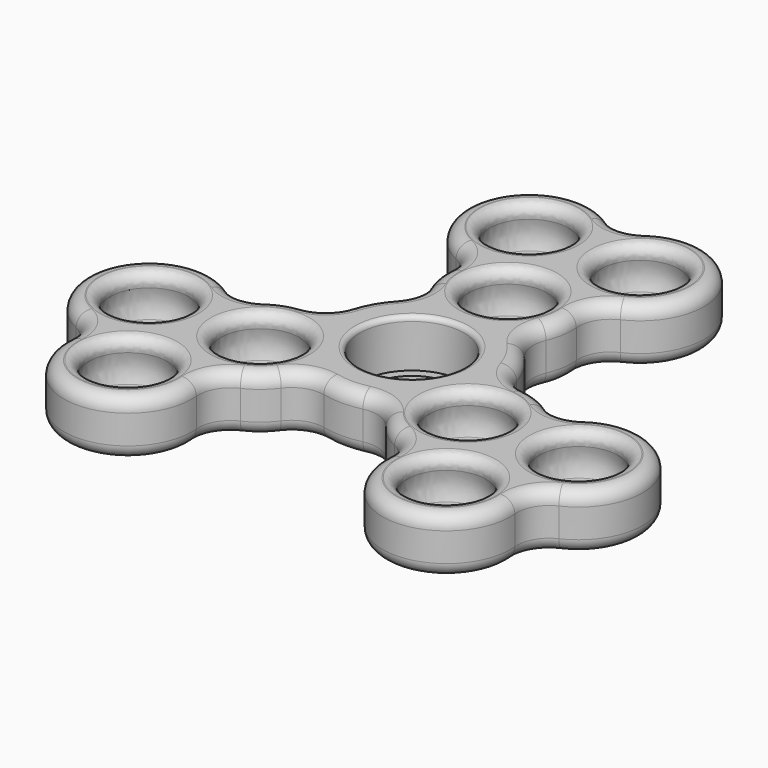
from build123d import *

# Parameters (mm, degrees)
F0_R      = 2.5
F0_R_2    = 6.525
F1_DEPTH  = 3.5
F2_DEPTH  = 3.5
F22_R     = 6.525
F22_R_2   = 5.3868073657
F23_DEPTH = 1
F24_R     = 1.7
F25_R     = 0.6
F26_R     = 1.32


with BuildPart() as f1:
    # F0 (on Top) → F1 (new body)
    with BuildSketch(Plane.XY):
        with BuildLine():
            ThreePointArc((62.7314133809, 3.8498463921), (61.4608563371, 1.9491717883), (59.3567896921, 1.0548660774))
            ThreePointArc((59.3567896921, 1.0548660774), (57.405087647, 0.5815289515), (55.6327668025, -0.3629644217))
            ThreePointArc((55.6327668025, -0.3629644217), (53.3233657257, -1.096978098), (51.0139646489, -0.3629644217))
            ThreePointArc((51.0139646489, -0.3629644217), (39.4669592652, -2.8949370692), (43.0477093227, -14.1609233929))
            ThreePointArc((43.0477093227, -14.1609233929), (44.8380843515, -15.7939165547), (45.3571103995, -18.1609233929))
            ThreePointArc((45.3571103995, -18.1609233929), (53.3233657257, -26.8949370692), (61.289621052, -18.1609233929))
            ThreePointArc((61.289621052, -18.1609233929), (61.8086470999, -15.7939165547), (63.5990221287, -14.1609233929))
            ThreePointArc((63.5990221287, -14.1609233929), (65.3031378059, -13.0982952045), (66.6889108041, -11.6447402157))
            ThreePointArc((66.6889108041, -11.6447402157), (68.5154355909, -10.2697179054), (70.796746604, -10.1197205304))
            ThreePointArc((70.796746604, -10.1197205304), (73.2419500127, -10.3949370692), (75.6871534215, -10.1197205304))
            ThreePointArc((75.6871534215, -10.1197205304), (77.9684644346, -10.2697179054), (79.7949892214, -11.6447402157))
            ThreePointArc((79.7949892214, -11.6447402157), (81.1807622196, -13.0982952045), (82.8848778968, -14.1609233929))
            ThreePointArc((82.8848778968, -14.1609233929), (84.6752529255, -15.7939165547), (85.1942789735, -18.1609233929))
            ThreePointArc((85.1942789735, -18.1609233929), (93.1605342998, -26.8949370692), (101.126789626, -18.1609233929))
            ThreePointArc((101.126789626, -18.1609233929), (101.645815674, -15.7939165547), (103.4361907028, -14.1609233929))
            ThreePointArc((103.4361907028, -14.1609233929), (107.0169407603, -2.8949370692), (95.4699353765, -0.3629644217))
            ThreePointArc((95.4699353765, -0.3629644217), (93.1605342998, -1.096978098), (90.851133223, -0.3629644217))
            ThreePointArc((90.851133223, -0.3629644217), (89.0788123785, 0.5815289515), (87.1271103334, 1.0548660774))
            ThreePointArc((87.1271103334, 1.0548660774), (85.0230436884, 1.9491717883), (83.7524866446, 3.8498463921))
            ThreePointArc((83.7524866446, 3.8498463921), (82.7682294544, 6.1050629308), (81.3072832359, 8.0850629308))
            ThreePointArc((81.3072832359, 8.0850629308), (80.2965292666, 10.1357349096), (80.5740711247, 12.4050629308))
            ThreePointArc((80.5740711247, 12.4050629308), (81.1400001716, 14.3319550455), (81.208205339, 16.3390766071))
            ThreePointArc((81.208205339, 16.3390766071), (81.727231387, 18.7060834453), (83.5176064158, 20.3390766071))
            ThreePointArc((83.5176064158, 20.3390766071), (87.0983564733, 31.6050629308), (75.5513510895, 34.1370355783))
            ThreePointArc((75.5513510895, 34.1370355783), (73.2419500127, 33.403021902), (70.932548936, 34.1370355783))
            ThreePointArc((70.932548936, 34.1370355783), (59.3855435522, 31.6050629308), (62.9662936097, 20.3390766071))
            ThreePointArc((62.9662936097, 20.3390766071), (64.7566686385, 18.7060834453), (65.2756946865, 16.3390766071))
            ThreePointArc((65.2756946865, 16.3390766071), (65.3438998539, 14.3319550455), (65.9098289008, 12.4050629308))
            ThreePointArc((65.9098289008, 12.4050629308), (66.1873707589, 10.1357349096), (65.1766167896, 8.0850629308))
            ThreePointArc((65.1766167896, 8.0850629308), (63.7156705711, 6.1050629308), (62.7314133809, 3.8498463921))
        make_face()
        with Locations((53.3233657257, -18.8949370692)):
            Circle(F0_R, mode=Mode.SUBTRACT)
        with Locations((46.3951624954, -6.8949370692)):
            Circle(F0_R, mode=Mode.SUBTRACT)
        with Locations((60.251568956, -6.8949370692)):
            Circle(F0_R, mode=Mode.SUBTRACT)
        with Locations((73.2419500127, 0.6050629308)):
            Circle(F0_R_2, mode=Mode.SUBTRACT)
        with Locations((93.1605342998, -18.8949370692)):
            Circle(F0_R, mode=Mode.SUBTRACT)
        with Locations((86.2323310695, -6.8949370692)):
            Circle(F0_R, mode=Mode.SUBTRACT)
        with Locations((100.0887375301, -6.8949370692)):
            Circle(F0_R, mode=Mode.SUBTRACT)
        with Locations((73.2419500127, 15.6050629308)):
            Circle(F0_R, mode=Mode.SUBTRACT)
        with Locations((66.3137467825, 27.6050629308)):
            Circle(F0_R, mode=Mode.SUBTRACT)
        with Locations((80.170153243, 27.6050629308)):
            Circle(F0_R, mode=Mode.SUBTRACT)
    extrude(amount=F1_DEPTH)

    # F0 (on Top) → F2 (join)
    with BuildSketch(Plane.XY):
        with BuildLine():
            ThreePointArc((62.7314133809, 3.8498463921), (61.4608563371, 1.9491717883), (59.3567896921, 1.0548660774))
            ThreePointArc((59.3567896921, 1.0548660774), (57.405087647, 0.5815289515), (55.6327668025, -0.3629644217))
            ThreePointArc((55.6327668025, -0.3629644217), (53.3233657257, -1.096978098), (51.0139646489, -0.3629644217))
            ThreePointArc((51.0139646489, -0.3629644217), (39.4669592652, -2.8949370692), (43.0477093227, -14.1609233929))
            ThreePointArc((43.0477093227, -14.1609233929), (44.8380843515, -15.7939165547), (45.3571103995, -18.1609233929))
            ThreePointArc((45.3571103995, -18.1609233929), (53.3233657257, -26.8949370692), (61.289621052, -18.1609233929))
            ThreePointArc((61.289621052, -18.1609233929), (61.8086470999, -15.7939165547), (63.5990221287, -14.1609233929))
            ThreePointArc((63.5990221287, -14.1609233929), (65.3031378059, -13.0982952045), (66.6889108041, -11.6447402157))
            ThreePointArc((66.6889108041, -11.6447402157), (68.5154355909, -10.2697179054), (70.796746604, -10.1197205304))
            ThreePointArc((70.796746604, -10.1197205304), (73.2419500127, -10.3949370692), (75.6871534215, -10.1197205304))
            ThreePointArc((75.6871534215, -10.1197205304), (77.9684644346, -10.2697179054), (79.7949892214, -11.6447402157))
            ThreePointArc((79.7949892214, -11.6447402157), (81.1807622196, -13.0982952045), (82.8848778968, -14.1609233929))
            ThreePointArc((82.8848778968, -14.1609233929), (84.6752529255, -15.7939165547), (85.1942789735, -18.1609233929))
            ThreePointArc((85.1942789735, -18.1609233929), (93.1605342998, -26.8949370692), (101.126789626, -18.1609233929))
            ThreePointArc((101.126789626, -18.1609233929), (101.645815674, -15.7939165547), (103.4361907028, -14.1609233929))
            ThreePointArc((103.4361907028, -14.1609233929), (107.0169407603, -2.8949370692), (95.4699353765, -0.3629644217))
            ThreePointArc((95.4699353765, -0.3629644217), (93.1605342998, -1.096978098), (90.851133223, -0.3629644217))
            ThreePointArc((90.851133223, -0.3629644217), (89.0788123785, 0.5815289515), (87.1271103334, 1.0548660774))
            ThreePointArc((87.1271103334, 1.0548660774), (85.0230436884, 1.9491717883), (83.7524866446, 3.8498463921))
            ThreePointArc((83.7524866446, 3.8498463921), (82.7682294544, 6.1050629308), (81.3072832359, 8.0850629308))
            ThreePointArc((81.3072832359, 8.0850629308), (80.2965292666, 10.1357349096), (80.5740711247, 12.4050629308))
            ThreePointArc((80.5740711247, 12.4050629308), (81.1400001716, 14.3319550455), (81.208205339, 16.3390766071))
            ThreePointArc((81.208205339, 16.3390766071), (81.727231387, 18.7060834453), (83.5176064158, 20.3390766071))
            ThreePointArc((83.5176064158, 20.3390766071), (87.0983564733, 31.6050629308), (75.5513510895, 34.1370355783))
            ThreePointArc((75.5513510895, 34.1370355783), (73.2419500127, 33.403021902), (70.932548936, 34.1370355783))
            ThreePointArc((70.932548936, 34.1370355783), (59.3855435522, 31.6050629308), (62.9662936097, 20.3390766071))
            ThreePointArc((62.9662936097, 20.3390766071), (64.7566686385, 18.7060834453), (65.2756946865, 16.3390766071))
            ThreePointArc((65.2756946865, 16.3390766071), (65.3438998539, 14.3319550455), (65.9098289008, 12.4050629308))
            ThreePointArc((65.9098289008, 12.4050629308), (66.1873707589, 10.1357349096), (65.1766167896, 8.0850629308))
            ThreePointArc((65.1766167896, 8.0850629308), (63.7156705711, 6.1050629308), (62.7314133809, 3.8498463921))
        make_face()
        with Locations((53.3233657257, -18.8949370692)):
            Circle(F0_R, mode=Mode.SUBTRACT)
        with Locations((46.3951624954, -6.8949370692)):
            Circle(F0_R, mode=Mode.SUBTRACT)
        with Locations((60.251568956, -6.8949370692)):
            Circle(F0_R, mode=Mode.SUBTRACT)
        with Locations((73.2419500127, 0.6050629308)):
            Circle(F0_R_2, mode=Mode.SUBTRACT)
        with Locations((93.1605342998, -18.8949370692)):
            Circle(F0_R, mode=Mode.SUBTRACT)
        with Locations((86.2323310695, -6.8949370692)):
            Circle(F0_R, mode=Mode.SUBTRACT)
        with Locations((100.0887375301, -6.8949370692)):
            Circle(F0_R, mode=Mode.SUBTRACT)
        with Locations((73.2419500127, 15.6050629308)):
            Circle(F0_R, mode=Mode.SUBTRACT)
        with Locations((66.3137467825, 27.6050629308)):
            Circle(F0_R, mode=Mode.SUBTRACT)
        with Locations((80.170153243, 27.6050629308)):
            Circle(F0_R, mode=Mode.SUBTRACT)
    extrude(amount=-F2_DEPTH)


with BuildPart() as f4:
    # F3 (on face) → F4 (revolve)
    with BuildSketch(Plane.XY):
        with BuildLine():
            Line((53.3233657257, -24.1249370692), (53.3233657257, -18.8949370692))
            Line((53.3233657257, -18.8949370692), (53.3233657257, -13.6649370692))
            ThreePointArc((53.3233657257, -13.6649370692), (48.0933657257, -18.8949370692), (53.3233657257, -24.1249370692))
        make_face()
    revolve(axis=Axis((53.3233657257, -16.2799370692, 0), (0, 1, 0)))


with BuildPart() as f7:
    # F6 (on face) → F7 (revolve)
    with BuildSketch(Plane.XY):
        with BuildLine():
            Line((93.1605342998, -24.1249370692), (93.1605342998, -18.8949370692))
            Line((93.1605342998, -18.8949370692), (93.1605342998, -13.6649370692))
            ThreePointArc((93.1605342998, -13.6649370692), (87.9305342998, -18.8949370692), (93.1605342998, -24.1249370692))
        make_face()
    revolve(axis=Axis((93.1605342998, -16.2799370692, 0), (0, 1, 0)))


with BuildPart() as f9:
    # F8 (on face) → F9 (revolve)
    with BuildSketch(Plane.XY):
        with BuildLine():
            Line((86.2323310695, -12.1249370692), (86.2323310695, -6.8949370692))
            Line((86.2323310695, -6.8949370692), (86.2323310695, -1.6649370692))
            ThreePointArc((86.2323310695, -1.6649370692), (81.0023310695, -6.8949370692), (86.2323310695, -12.1249370692))
        make_face()
    revolve(axis=Axis((86.2323310695, -4.2799370692, 0), (0, 1, 0)))


with BuildPart() as f11:
    # F10 (on face) → F11 (revolve)
    with BuildSketch(Plane.XY):
        with BuildLine():
            Line((100.0887375301, -12.1249370692), (100.0887375301, -6.8949370692))
            Line((100.0887375301, -6.8949370692), (100.0887375301, -1.6649370692))
            ThreePointArc((100.0887375301, -1.6649370692), (94.8587375301, -6.8949370692), (100.0887375301, -12.1249370692))
        make_face()
    revolve(axis=Axis((100.0887375301, -9.5099370692, 0), (0, -1, 0)))


with BuildPart() as f13:
    # F12 (on face) → F13 (revolve)
    with BuildSketch(Plane.XY):
        with BuildLine():
            Line((73.2419500127, 10.3750629308), (73.2419500127, 15.6050629308))
            Line((73.2419500127, 15.6050629308), (73.2419500127, 20.8350629308))
            ThreePointArc((73.2419500127, 20.8350629308), (68.0119500127, 15.6050629308), (73.2419500127, 10.3750629308))
        make_face()
    revolve(axis=Axis((73.2419500127, 12.9900629308, 0), (0, -1, 0)))


with BuildPart() as f15:
    # F14 (on face) → F15 (revolve)
    with BuildSketch(Plane.XY):
        with BuildLine():
            Line((66.3137467825, 22.3550629308), (66.3137467825, 27.6050629308))
            Line((66.3137467825, 27.6050629308), (66.3137467825, 32.8550629308))
            ThreePointArc((66.3137467825, 32.8550629308), (61.0637467825, 27.6050629308), (66.3137467825, 22.3550629308))
        make_face()
    revolve(axis=Axis((66.3137467825, 24.9800629308, 0), (0, -1, 0)))


with BuildPart() as f17:
    # F5 (on face) → F17 (revolve)
    with BuildSketch(Plane.XY):
        with BuildLine():
            Line((60.251568956, -12.1449370692), (60.251568956, -6.8949370692))
            Line((60.251568956, -6.8949370692), (60.251568956, -1.6449370692))
            ThreePointArc((60.251568956, -1.6449370692), (55.001568956, -6.8949370692), (60.251568956, -12.1449370692))
        make_face()
    revolve(axis=Axis((60.251568956, -4.2699370692, 0), (0, 1, 0)))


with BuildPart() as f18:
    # F16 (on face) → F18 (revolve)
    with BuildSketch(Plane.XY):
        with BuildLine():
            Line((80.170153243, 22.3750629308), (80.170153243, 27.6050629308))
            Line((80.170153243, 27.6050629308), (80.170153243, 32.8350629308))
            ThreePointArc((80.170153243, 32.8350629308), (74.940153243, 27.6050629308), (80.170153243, 22.3750629308))
        make_face()
    revolve(axis=Axis((80.170153243, 24.9900629308, 0), (0, -1, 0)))


with BuildPart() as f20:
    # F19 (on face) → F20 (revolve)
    with BuildSketch(Plane.XY):
        with BuildLine():
            Line((46.3951624954, -12.1249370692), (46.3951624954, -6.8949370692))
            Line((46.3951624954, -6.8949370692), (46.3951624954, -1.6649370692))
            ThreePointArc((46.3951624954, -1.6649370692), (41.1651624954, -6.8949370692), (46.3951624954, -12.1249370692))
        make_face()
    revolve(axis=Axis((46.3951624954, -9.5099370692, 0), (0, -1, 0)))


with BuildPart() as f1_1:
    add(f1.part)

    # F21: cut F15, F18, F13, F9, F11, F20, F17, F4, F7
    add(f15.part, mode=Mode.SUBTRACT)
    add(f18.part, mode=Mode.SUBTRACT)
    add(f13.part, mode=Mode.SUBTRACT)
    add(f9.part, mode=Mode.SUBTRACT)
    add(f11.part, mode=Mode.SUBTRACT)
    add(f20.part, mode=Mode.SUBTRACT)
    add(f17.part, mode=Mode.SUBTRACT)
    add(f4.part, mode=Mode.SUBTRACT)
    add(f7.part, mode=Mode.SUBTRACT)

    # F22 (on face) → F23 (join)
    with BuildSketch(Plane(origin=(0, 0, -3.5), x_dir=(1, 0, 0), z_dir=(0, 0, -1))):
        with Locations((73.2419500127, -0.6050629308)):
            Circle(F22_R)
        with Locations((73.2419500127, -0.6050629308)):
            Circle(F22_R_2, mode=Mode.SUBTRACT)
    extrude(amount=-F23_DEPTH)

    # F24
    f24_edges = [f1_1.edges().sort_by_distance(p)[0] for p in [
        (87.098356, 31.605063, 3.5),
        (87.098356, 31.605063, -3.5),
        (66.187371, 10.135735, 3.5),
        (66.187371, 10.135735, -3.5),
        (65.3439, 14.331955, 3.5),
        (65.3439, 14.331955, -3.5),
        (63.715671, 6.105063, 3.5),
        (64.756669, 18.706083, 3.5),
        (61.460856, 1.949172, 3.5),
        (59.385544, 31.605063, 3.5),
        (57.405088, 0.581529, 3.5),
        (73.24195, 33.403022, 3.5),
        (53.323366, -1.096978, 3.5),
        (39.466959, -2.894937, 3.5),
        (81.727231, 18.706083, 3.5),
        (44.838084, -15.793917, 3.5),
        (81.14, 14.331955, 3.5),
        (53.323366, -26.894937, 3.5),
        (80.296529, 10.135735, 3.5),
        (61.808647, -15.793917, 3.5),
        (82.768229, 6.105063, 3.5),
        (65.303138, -13.098295, 3.5),
        (85.023044, 1.949172, 3.5),
        (68.515436, -10.269718, 3.5),
        (89.078812, 0.581529, 3.5),
        (73.24195, -10.394937, 3.5),
        (93.160534, -1.096978, 3.5),
        (77.968464, -10.269718, 3.5),
        (107.016941, -2.894937, 3.5),
        (81.180762, -13.098295, 3.5),
        (101.645816, -15.793917, 3.5),
        (84.675253, -15.793917, 3.5),
        (93.160534, -26.894937, 3.5),
        (63.715671, 6.105063, -3.5),
        (61.460856, 1.949172, -3.5),
        (57.405088, 0.581529, -3.5),
        (53.323366, -1.096978, -3.5),
        (39.466959, -2.894937, -3.5),
        (44.838084, -15.793917, -3.5),
        (53.323366, -26.894937, -3.5),
        (61.808647, -15.793917, -3.5),
        (65.303138, -13.098295, -3.5),
        (68.515436, -10.269718, -3.5),
        (73.24195, -10.394937, -3.5),
        (77.968464, -10.269718, -3.5),
        (81.180762, -13.098295, -3.5),
        (84.675253, -15.793917, -3.5),
        (93.160534, -26.894937, -3.5),
        (101.645816, -15.793917, -3.5),
        (107.016941, -2.894937, -3.5),
        (93.160534, -1.096978, -3.5),
        (89.078812, 0.581529, -3.5),
        (85.023044, 1.949172, -3.5),
        (82.768229, 6.105063, -3.5),
        (80.296529, 10.135735, -3.5),
        (81.14, 14.331955, -3.5),
        (81.727231, 18.706083, -3.5),
        (73.24195, 33.403022, -3.5),
        (59.385544, 31.605063, -3.5),
        (64.756669, 18.706083, -3.5),
    ]]
    fillet(f24_edges, radius=F24_R)

    # F25
    f25_edges = [f1_1.edges().sort_by_distance(p)[0] for p in [
        (66.71695, 0.605063, 3.5),
    ]]
    fillet(f25_edges, radius=F25_R)

    # F26
    f26_edges = [f1_1.edges().sort_by_distance(p)[0] for p in [
        (93.160534, -15.008692, 3.5),
        (86.232331, -3.008692, 3.5),
        (100.088738, -3.008692, 3.5),
        (53.323366, -15.008692, 3.5),
        (46.395162, -3.008692, 3.5),
        (60.251569, -2.981818, 3.5),
        (73.24195, 19.491308, 3.5),
        (66.313747, 31.518182, 3.5),
        (80.170153, 31.491308, 3.5),
        (53.323366, -15.008692, -3.5),
        (46.395162, -3.008692, -3.5),
        (60.251569, -2.981818, -3.5),
        (86.232331, -3.008692, -3.5),
        (93.160534, -15.008692, -3.5),
        (100.088738, -3.008692, -3.5),
        (73.24195, 19.491308, -3.5),
        (80.170153, 31.491308, -3.5),
        (66.313747, 31.518182, -3.5),
    ]]
    fillet(f26_edges, radius=F26_R)


solid = f1_1.part
